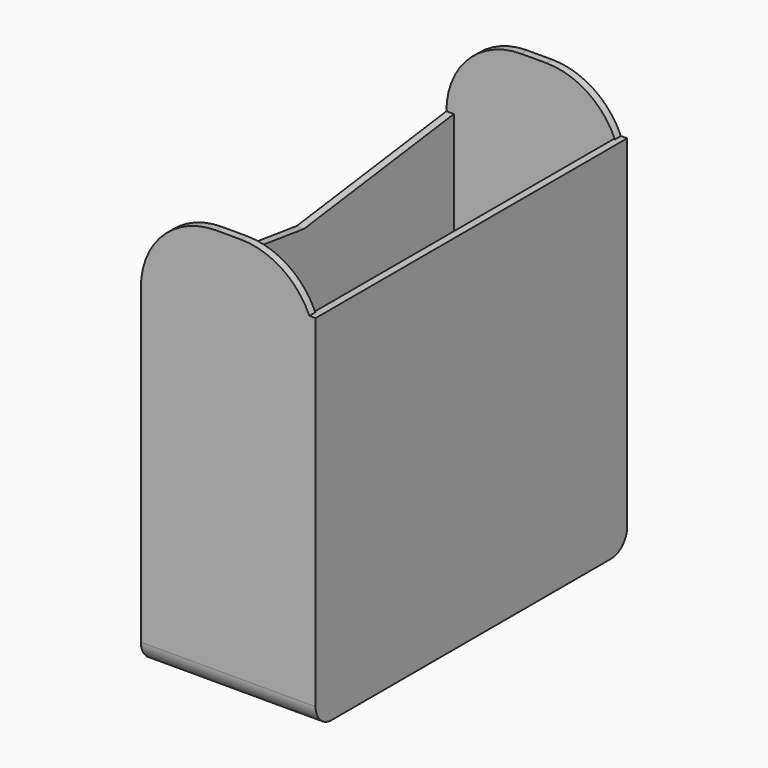
from build123d import *

# Parameters (mm, degrees)
F1_DEPTH  = 35
F2_R      = 30
F5_DEPTH  = 3
F8_DEPTH  = 3
F10_DEPTH = 2
F11_R     = 1.999


# Not quite as in the source:
# - a fillet or chamfer is up to 0.001 mm smaller than in the source, because OpenCascade refuses the exact size


with BuildPart() as f1:
    # F0 (on Right) → F1 (new body, symmetric)
    with BuildSketch(Plane.YZ):
        with BuildLine():
            Line((-75, 163), (-78, 163))
            Line((-78, 163), (-78, 8))
            ThreePointArc((-78, 8), (-75.6568542495, 2.3431457505), (-70, 0))
            Line((-70, 0), (0, 0))
            Line((0, 0), (0, 3))
            Line((0, 3), (-67, 3))
            ThreePointArc((-67, 3), (-72.6568542495, 5.3431457505), (-75, 11))
            Line((-75, 11), (-75, 163))
        make_face()
        with BuildLine():
            Line((0, 3), (0, 0))
            Line((0, 0), (70, 0))
            ThreePointArc((70, 0), (75.6568542495, 2.3431457505), (78, 8))
            Line((78, 8), (78, 163))
            Line((78, 163), (75, 163))
            Line((75, 163), (75, 11))
            ThreePointArc((75, 11), (72.6568542495, 5.3431457505), (67, 3))
            Line((67, 3), (0, 3))
        make_face()
    extrude(amount=F1_DEPTH, both=True)

    # F2
    f2_edges = [f1.edges().sort_by_distance(p)[0] for p in [
        (35, -76.5, 163),
        (35, 76.5, 163),
        (-35, 76.5, 163),
        (-35, -76.5, 163),
    ]]
    fillet(f2_edges, radius=F2_R)

    # F4 (on offset) → F5 (join)
    with BuildSketch(Plane(origin=(-35, 0, 0), x_dir=(0, -1, 0), z_dir=(-1, 0, 0))):
        with BuildLine():
            Line((-75, 133), (-78, 133))
            Line((-78, 133), (-78, 8))
            ThreePointArc((-78, 8), (-75.6568542495, 2.3431457505), (-70, 0))
            Line((-70, 0), (0, 0))
            Line((0, 0), (70, 0))
            ThreePointArc((70, 0), (75.6568542495, 2.3431457505), (78, 8))
            Line((78, 8), (78, 133))
            Line((78, 133), (75, 133))
            Line((75, 133), (0, 123))
            Line((0, 123), (-75, 133))
        make_face()
    extrude(amount=-F5_DEPTH)

    # F7 (on offset) → F8 (join)
    with BuildSketch(Plane.YZ.offset(35)):
        with BuildLine():
            Line((-78, 145), (-78, 8))
            ThreePointArc((-78, 8), (-75.6568542495, 2.3431457505), (-70, 0))
            Line((-70, 0), (0, 0))
            Line((0, 0), (70, 0))
            ThreePointArc((70, 0), (75.6568542495, 2.3431457505), (78, 8))
            Line((78, 8), (78, 145))
            Line((78, 145), (0, 145))
            Line((0, 145), (-78, 145))
        make_face()
    extrude(amount=-F8_DEPTH)

    # F9 (on offset) → F10 (join)
    with BuildSketch(Plane(origin=(-35, 0, 0), x_dir=(0, -1, 0), z_dir=(-1, 0, 0))):
        with BuildLine():
            add(Edge.make_bspline(
                [(22.5, 95), (22.5, 116.6506350946), (-11.25, 105.8253175473), (-45, 95), (-11.25, 84.1746824527), (22.5, 73.3493649054), (22.5, 95)],
                knots=[0, 0, 0, 2.0943951024, 2.0943951024, 4.1887902048, 4.1887902048, 6.2831853072, 6.2831853072, 6.2831853072], degree=2, weights=[1, 0.5, 1, 0.5, 1, 0.5, 1]))
        make_face()
    extrude(amount=F10_DEPTH)

    # F11 (radius 2 in the source; OpenCascade refuses exactly that, so slightly less here)
    f11_edges = [f1.edges().sort_by_distance(p)[0] for p in [
        (-37, 22.5, 95.000001),
    ]]
    fillet(f11_edges, radius=F11_R)


solid = f1.part
